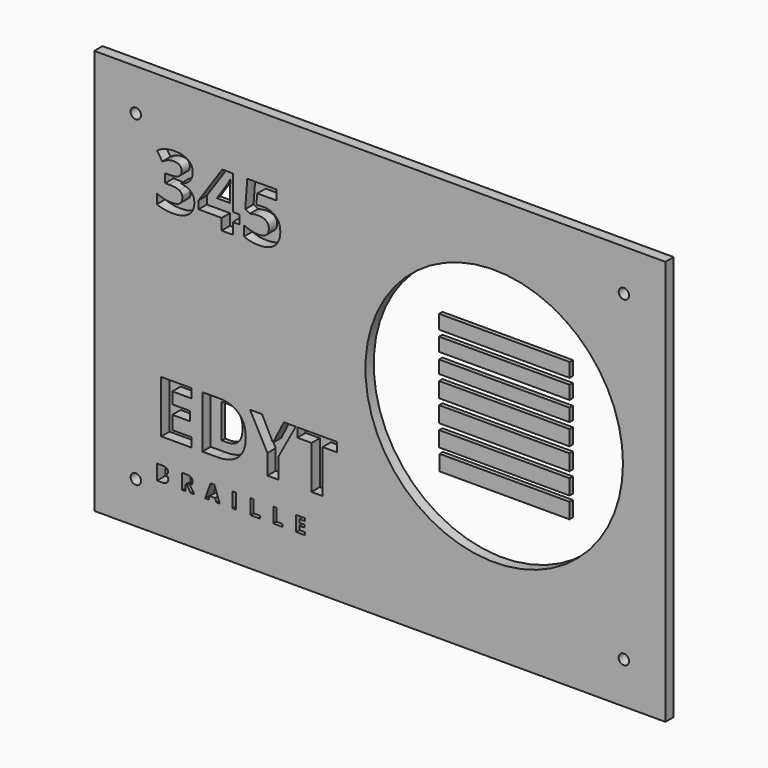
from build123d import *

# Parameters (mm, degrees)
F0_W           = 349.25
F0_H           = 247.65
F0_R           = 3.175
F0_W_2         = 1.9502034897
F0_H_2         = 9.195541532
F0_R_2         = 78.7423234547
F1_DEPTH       = 6.35
F0_W_3         = 79.7690153122
F0_H_3         = 8.5733048618
F0_H_4         = 8.2005523145
F0_H_5         = 7.8277997673
F0_H_6         = 9.3188099563
F0_H_7         = 9.6915662289
F0_H_8         = 9.3188136816
F0_W_4         = 79.3962478638
F0_H_9         = 9.4509058177
F0_TEXT_SIZE   = 44.8574507982
F0_TEXT_SIZE_2 = 46.3020833333
F2_DEPTH       = 2.54


# Not quite as in the source:
# - Text() gives the source's letters only with a copy of the font that has no kerning and outlines rounded to 1/6400 em; it was checked with that copy


with BuildPart() as f1:
    # F0 (on Front) → F1 (new body)
    with BuildSketch(Plane.XZ):
        with Locations((111.7297765017, -62.4566947639)):
            Rectangle(F0_W, F0_H)
        with Locations((-37.4952234983, -160.8816947639)):
            Circle(F0_R, mode=Mode.SUBTRACT)
        with BuildLine():
            Line((-24.4460603303, -157.455727458), (-24.4460603303, -148.260185926))
            Line((-24.4460603303, -148.260185926), (-21.5841518036, -148.260185926))
            add(Edge.make_bspline(
                [(-21.5841518036, -148.260185926), (-19.6279105322, -148.260185926), (-18.7443818098, -148.8166681395)],
                knots=[0, 0, 0, 1, 1, 1], degree=2))
            add(Edge.make_bspline(
                [(-18.7443818098, -148.8166681395), (-17.8608530874, -149.3731503531), (-17.8608530874, -150.5867444752)],
                knots=[0, 0, 0, 1, 1, 1], degree=2))
            add(Edge.make_bspline(
                [(-17.8608530874, -150.5867444752), (-17.8608530874, -151.4119079744), (-18.2472711163, -151.9402138733)],
                knots=[0, 0, 0, 1, 1, 1], degree=2))
            add(Edge.make_bspline(
                [(-18.2472711163, -151.9402138733), (-18.6336891453, -152.4685197722), (-19.2757065996, -152.575187249)],
                knots=[0, 0, 0, 1, 1, 1], degree=2))
            Line((-19.2757065996, -152.575187249), (-19.2757065996, -152.6375776599))
            add(Edge.make_bspline(
                [(-19.2757065996, -152.6375776599), (-18.4022408467, -152.8327992683), (-18.0148165208, -153.3671429489)],
                knots=[0, 0, 0, 1, 1, 1], degree=2))
            add(Edge.make_bspline(
                [(-18.0148165208, -153.3671429489), (-17.6273921949, -153.9014866295), (-17.6273921949, -154.7890405397)],
                knots=[0, 0, 0, 1, 1, 1], degree=2))
            add(Edge.make_bspline(
                [(-17.6273921949, -154.7890405397), (-17.6273921949, -156.0469117276), (-18.537084638, -156.7513195928)],
                knots=[0, 0, 0, 1, 1, 1], degree=2))
            add(Edge.make_bspline(
                [(-18.537084638, -156.7513195928), (-19.4467770811, -157.455727458), (-21.0065373541, -157.455727458)],
                knots=[0, 0, 0, 1, 1, 1], degree=2))
            Line((-21.0065373541, -157.455727458), (-24.4460603303, -157.455727458))
        make_face(mode=Mode.SUBTRACT)
        with BuildLine():
            Line((-6.1113298955, -153.9276503502), (-7.1478157544, -153.9276503502))
            Line((-7.1478157544, -153.9276503502), (-7.1478157544, -157.455727458))
            Line((-7.1478157544, -157.455727458), (-9.0980192441, -157.455727458))
            Line((-9.0980192441, -157.455727458), (-9.0980192441, -148.260185926))
            Line((-9.0980192441, -148.260185926), (-6.4192567623, -148.260185926))
            add(Edge.make_bspline(
                [(-6.4192567623, -148.260185926), (-4.543519247, -148.260185926), (-3.6448960703, -148.9424552583)],
                knots=[0, 0, 0, 1, 1, 1], degree=2))
            add(Edge.make_bspline(
                [(-3.6448960703, -148.9424552583), (-2.7462728937, -149.6247245907), (-2.7462728937, -151.015426976)],
                knots=[0, 0, 0, 1, 1, 1], degree=2))
            add(Edge.make_bspline(
                [(-2.7462728937, -151.015426976), (-2.7462728937, -151.8265023179), (-3.1920624427, -152.4584568027)],
                knots=[0, 0, 0, 1, 1, 1], degree=2))
            add(Edge.make_bspline(
                [(-3.1920624427, -152.4584568027), (-3.6378519917, -153.0904112875), (-4.4569777092, -153.4486530018)],
                knots=[0, 0, 0, 1, 1, 1], degree=2))
            add(Edge.make_bspline(
                [(-4.4569777092, -153.4486530018), (-2.3799808038, -156.5500602027), (-1.7520515068, -157.455727458)],
                knots=[0, 0, 0, 1, 1, 1], degree=2))
            Line((-1.7520515068, -157.455727458), (-3.91558995, -157.455727458))
            Line((-3.91558995, -157.455727458), (-6.1113298955, -153.9276503502))
        make_face(mode=Mode.SUBTRACT)
        Polygon((13.8294504719, -157.455727458), (11.7283024396, -157.455727458), (11.0621338585, -155.2660252941), (7.7091524201, -155.2660252941), (7.042983839, -157.455727458), (4.9418358067, -157.455727458), (8.1881497684, -148.2219466419), (10.5710609468, -148.2219466419), align=None, mode=Mode.SUBTRACT)
        with Locations((22.6556810231, -152.857956692)):
            Rectangle(F0_W_2, F0_H_2, mode=Mode.SUBTRACT)
        Polygon((38.3186930548, -157.455727458), (32.6391530672, -157.455727458), (32.6391530672, -148.260185926), (34.5893565569, -148.260185926), (34.5893565569, -155.8456523375), (38.3186930548, -155.8456523375), align=None, mode=Mode.SUBTRACT)
        Polygon((52.2901199129, -157.455727458), (46.6105799254, -157.455727458), (46.6105799254, -148.260185926), (48.5607834151, -148.260185926), (48.5607834151, -155.8456523375), (52.2901199129, -155.8456523375), align=None, mode=Mode.SUBTRACT)
        Polygon((65.8771413361, -155.8456523375), (65.8771413361, -157.455727458), (60.5820067835, -157.455727458), (60.5820067835, -148.260185926), (65.8771413361, -148.260185926), (65.8771413361, -149.8581854831), (62.5322102732, -149.8581854831), (62.5322102732, -151.8768171655), (65.6456930375, -151.8768171655), (65.6456930375, -153.4748167226), (62.5322102732, -153.4748167226), (62.5322102732, -155.8456523375), align=None, mode=Mode.SUBTRACT)
        Polygon((-3.5052732486, -127.2468779888), (-3.5052732486, -132.8540593386), (-21.9458909126, -132.8540593386), (-21.9458909126, -100.8300448547), (-3.5052732486, -100.8300448547), (-3.5052732486, -106.3951723443), (-15.1541925027, -106.3951723443), (-15.1541925027, -113.4251759616), (-4.3113055676, -113.4251759616), (-4.3113055676, -118.9903034513), (-15.1541925027, -118.9903034513), (-15.1541925027, -127.2468779888), align=None, mode=Mode.SUBTRACT)
        with BuildLine():
            add(Edge.make_bspline(
                [(25.4067555862, -104.9688455885), (29.7453121556, -109.1076463223), (29.7453121556, -116.5371616107)],
                knots=[0, 0, 0, 1, 1, 1], degree=2))
            add(Edge.make_bspline(
                [(29.7453121556, -116.5371616107), (29.7453121556, -124.4432873139), (25.242044634, -128.6486733262)],
                knots=[0, 0, 0, 1, 1, 1], degree=2))
            add(Edge.make_bspline(
                [(25.242044634, -128.6486733262), (20.7387771125, -132.8540593386), (12.2438973676, -132.8540593386)],
                knots=[0, 0, 0, 1, 1, 1], degree=2))
            Line((12.2438973676, -132.8540593386), (3.1742815344, -132.8540593386))
            Line((3.1742815344, -132.8540593386), (3.1742815344, -100.8300448547))
            Line((3.1742815344, -100.8300448547), (13.2251541038, -100.8300448547))
            add(Edge.make_bspline(
                [(13.2251541038, -100.8300448547), (21.0681990168, -100.8300448547), (25.4067555862, -104.9688455885)],
                knots=[0, 0, 0, 1, 1, 1], degree=2))
        make_face(mode=Mode.SUBTRACT)
        Polygon((39.7120770048, -100.8300448547), (46.3495779276, -114.0139300033), (53.0291327105, -100.8300448547), (60.3465043719, -100.8300448547), (49.7208957141, -120.3920987887), (49.7208957141, -132.8540593386), (42.978260141, -132.8540593386), (42.978260141, -120.609377066), (32.3526514832, -100.8300448547), align=None, mode=Mode.SUBTRACT)
        Polygon((76.7334918666, -106.4792800646), (76.7334918666, -132.8540593386), (69.9417934567, -132.8540593386), (69.9417934567, -106.4792800646), (61.2436533879, -106.4792800646), (61.2436533879, -100.8300448547), (85.4246229588, -100.8300448547), (85.4246229588, -106.4792800646), align=None, mode=Mode.SUBTRACT)
        with Locations((260.9547765017, -160.8816947639)):
            Circle(F0_R, mode=Mode.SUBTRACT)
        with BuildLine():
            add(Edge.make_bspline(
                [(-5.6503231396, 21.3764310499), (-2.6768612256, 19.2964546502), (-2.6768612256, 15.5922879835)],
                knots=[0, 0, 0, 1, 1, 1], degree=2))
            add(Edge.make_bspline(
                [(-2.6768612256, 15.5922879835), (-2.6768612256, 12.4958361606), (-4.5542660107, 10.3254260043)],
                knots=[0, 0, 0, 1, 1, 1], degree=2))
            add(Edge.make_bspline(
                [(-4.5542660107, 10.3254260043), (-6.4316707959, 8.1550158481), (-9.8247453401, 7.3374946892)],
                knots=[0, 0, 0, 1, 1, 1], degree=2))
            Line((-9.8247453401, 7.3374946892), (-9.8247453401, 7.2072700799))
            add(Edge.make_bspline(
                [(-9.8247453401, 7.2072700799), (-5.8167212516, 6.7080757439), (-3.7620663037, 4.7727933546)],
                knots=[0, 0, 0, 1, 1, 1], degree=2))
            add(Edge.make_bspline(
                [(-3.7620663037, 4.7727933546), (-1.7074113558, 2.8375109653), (-1.7074113558, -0.4398083707)],
                knots=[0, 0, 0, 1, 1, 1], degree=2))
            add(Edge.make_bspline(
                [(-1.7074113558, -0.4398083707), (-1.7074113558, -5.2074760139), (-5.1655982047, -7.8662284553)],
                knots=[0, 0, 0, 1, 1, 1], degree=2))
            add(Edge.make_bspline(
                [(-5.1655982047, -7.8662284553), (-8.6237850537, -10.5249808967), (-15.0409644157, -10.5249808967)],
                knots=[0, 0, 0, 1, 1, 1], degree=2))
            add(Edge.make_bspline(
                [(-15.0409644157, -10.5249808967), (-20.4235816032, -10.5249808967), (-24.5835344026, -8.7380098681)],
                knots=[0, 0, 0, 1, 1, 1], degree=2))
            Line((-24.5835344026, -8.7380098681), (-24.5835344026, -2.7910860399))
            add(Edge.make_bspline(
                [(-24.5835344026, -2.7910860399), (-22.6663387646, -3.7605359097), (-20.3584692985, -4.3718681037)],
                knots=[0, 0, 0, 1, 1, 1], degree=2))
            add(Edge.make_bspline(
                [(-20.3584692985, -4.3718681037), (-18.0505998323, -4.9832002978), (-15.7933732698, -4.9832002978)],
                knots=[0, 0, 0, 1, 1, 1], degree=2))
            add(Edge.make_bspline(
                [(-15.7933732698, -4.9832002978), (-12.3279517204, -4.9832002978), (-10.6784400016, -3.8075614631)],
                knots=[0, 0, 0, 1, 1, 1], degree=2))
            add(Edge.make_bspline(
                [(-10.6784400016, -3.8075614631), (-9.0289282829, -2.6319226285), (-9.0289282829, -0.027430441)],
                knots=[0, 0, 0, 1, 1, 1], degree=2))
            add(Edge.make_bspline(
                [(-9.0289282829, -0.027430441), (-9.0289282829, 2.2949084262), (-10.9280371696, 3.2679756463)],
                knots=[0, 0, 0, 1, 1, 1], degree=2))
            add(Edge.make_bspline(
                [(-10.9280371696, 3.2679756463), (-12.8271460563, 4.2410428663), (-16.9870988558, 4.2410428663)],
                knots=[0, 0, 0, 1, 1, 1], degree=2))
            Line((-16.9870988558, 4.2410428663), (-19.4975399365, 4.2410428663))
            Line((-19.4975399365, 4.2410428663), (-19.4975399365, 9.6019559522))
            Line((-19.4975399365, 9.6019559522), (-16.9436906526, 9.6019559522))
            add(Edge.make_bspline(
                [(-16.9436906526, 9.6019559522), (-13.1020646761, 9.6019559522), (-11.3259456982, 10.6075793246)],
                knots=[0, 0, 0, 1, 1, 1], degree=2))
            add(Edge.make_bspline(
                [(-11.3259456982, 10.6075793246), (-9.5498267204, 11.613202697), (-9.5498267204, 14.0512967726)],
                knots=[0, 0, 0, 1, 1, 1], degree=2))
            add(Edge.make_bspline(
                [(-9.5498267204, 14.0512967726), (-9.5498267204, 17.8061063429), (-14.2523820589, 17.8061063429)],
                knots=[0, 0, 0, 1, 1, 1], degree=2))
            add(Edge.make_bspline(
                [(-14.2523820589, 17.8061063429), (-15.8801896761, 17.8061063429), (-17.5658748974, 17.2635038038)],
                knots=[0, 0, 0, 1, 1, 1], degree=2))
            add(Edge.make_bspline(
                [(-17.5658748974, 17.2635038038), (-19.2515601188, 16.7209012647), (-21.3062150667, 15.3897163689)],
                knots=[0, 0, 0, 1, 1, 1], degree=2))
            Line((-21.3062150667, 15.3897163689), (-24.5401261995, 20.2007922153))
            add(Edge.make_bspline(
                [(-24.5401261995, 20.2007922153), (-20.018438374, 23.4564074496), (-13.753187723, 23.4564074496)],
                knots=[0, 0, 0, 1, 1, 1], degree=2))
            add(Edge.make_bspline(
                [(-13.753187723, 23.4564074496), (-8.6237850537, 23.4564074496), (-5.6503231396, 21.3764310499)],
                knots=[0, 0, 0, 1, 1, 1], degree=2))
        make_face(mode=Mode.SUBTRACT)
        Polygon((25.7844506234, 2.20809202), (25.7844506234, -3.2179333707), (21.8053653369, -3.2179333707), (21.8053653369, -10.0691947639), (14.9758080453, -10.0691947639), (14.9758080453, -3.2179333707), (0.8681420296, -3.2179333707), (0.8681420296, 1.6437853793), (15.3664818734, 22.9861519158), (21.8053653369, 22.9861519158), (21.8053653369, 2.20809202), align=None, mode=Mode.SUBTRACT)
        with Locations((-37.4952234983, 35.9683052361)):
            Circle(F0_R, mode=Mode.SUBTRACT)
        with BuildLine():
            add(Edge.make_bspline(
                [(36.9765323291, 10.7305692335), (38.3583601286, 11.0488960564), (40.391310975, 11.0488960564)],
                knots=[0, 0, 0, 1, 1, 1], degree=2))
            add(Edge.make_bspline(
                [(40.391310975, 11.0488960564), (45.1806827197, 11.0488960564), (48.0203026742, 8.3575874627)],
                knots=[0, 0, 0, 1, 1, 1], degree=2))
            add(Edge.make_bspline(
                [(48.0203026742, 8.3575874627), (50.8599226286, 5.6662788689), (50.8599226286, 0.9854276319)],
                knots=[0, 0, 0, 1, 1, 1], degree=2))
            add(Edge.make_bspline(
                [(50.8599226286, 0.9854276319), (50.8599226286, -4.5491182665), (47.4451439828, -7.5370495816)],
                knots=[0, 0, 0, 1, 1, 1], degree=2))
            add(Edge.make_bspline(
                [(47.4451439828, -7.5370495816), (44.0303653369, -10.5249808967), (37.6782982796, -10.5249808967)],
                knots=[0, 0, 0, 1, 1, 1], degree=2))
            add(Edge.make_bspline(
                [(37.6782982796, -10.5249808967), (32.1582217822, -10.5249808967), (28.7723819385, -8.7380098681)],
                knots=[0, 0, 0, 1, 1, 1], degree=2))
            Line((28.7723819385, -8.7380098681), (28.7723819385, -2.6970349332))
            add(Edge.make_bspline(
                [(28.7723819385, -2.6970349332), (30.5521182666, -3.6447807014), (32.9287173877, -4.2452608446)],
                knots=[0, 0, 0, 1, 1, 1], degree=2))
            add(Edge.make_bspline(
                [(32.9287173877, -4.2452608446), (35.3053165088, -4.8457409879), (37.4250837614, -4.8457409879)],
                knots=[0, 0, 0, 1, 1, 1], degree=2))
            add(Edge.make_bspline(
                [(37.4250837614, -4.8457409879), (43.8277937224, -4.8457409879), (43.8277937224, 0.3994168897)],
                knots=[0, 0, 0, 1, 1, 1], degree=2))
            add(Edge.make_bspline(
                [(43.8277937224, 0.3994168897), (43.8277937224, 5.3985949496), (37.2008080453, 5.3985949496)],
                knots=[0, 0, 0, 1, 1, 1], degree=2))
            add(Edge.make_bspline(
                [(37.2008080453, 5.3985949496), (36.0070824593, 5.3985949496), (34.5601423552, 5.1598498325)],
                knots=[0, 0, 0, 1, 1, 1], degree=2))
            add(Edge.make_bspline(
                [(34.5601423552, 5.1598498325), (33.113202251, 4.9211047153), (32.2088646859, 4.6461860955)],
                knots=[0, 0, 0, 1, 1, 1], degree=2))
            Line((32.2088646859, 4.6461860955), (29.4235049854, 6.1437691033))
            Line((29.4235049854, 6.1437691033), (30.667873475, 22.9861519158))
            Line((30.667873475, 22.9861519158), (48.5954613656, 22.9861519158))
            Line((48.5954613656, 22.9861519158), (48.5954613656, 17.0609321892))
            Line((48.5954613656, 17.0609321892), (36.7956648161, 17.0609321892))
            Line((36.7956648161, 17.0609321892), (36.1879499724, 10.571405822))
            Line((36.1879499724, 10.571405822), (36.9765323291, 10.7305692335))
        make_face(mode=Mode.SUBTRACT)
        with Locations((181.6470623016, -55.6943193078)):
            Circle(F0_R_2, mode=Mode.SUBTRACT)
        with Locations((260.9547765017, 35.9683052361)):
            Circle(F0_R, mode=Mode.SUBTRACT)
    extrude(amount=F1_DEPTH)


with BuildPart() as f2:
    # F0 (on Front) → F2 (new body)
    with BuildSketch(Plane.XZ):
        with Locations((182.7652901411, -20.0964603573)):
            Rectangle(F0_W_3, F0_H_3)
        with Locations((182.7652901411, -32.2109144181)):
            Rectangle(F0_W_3, F0_H_4)
        with Locations((182.7652901411, -44.3253684789)):
            Rectangle(F0_W_3, F0_H_5)
        with Locations((182.7652901411, -56.626195088)):
            Rectangle(F0_W_3, F0_H_6)
        with Locations((182.7652901411, -69.8589086533)):
            Rectangle(F0_W_3, F0_H_7)
        with Locations((182.7652901411, -83.0916166306)):
            Rectangle(F0_W_3, F0_H_8)
        with Locations((182.9516738653, -95.831241855)):
            Rectangle(F0_W_4, F0_H_9)
        with Locations((-25.9760525078, -132.8540593386)):
            Text('EDYT', F0_TEXT_SIZE, font='Open Sans', font_style=FontStyle.BOLD, text_align=(TextAlign.LEFT, TextAlign.BOTTOM))
        with Locations((-26.3488013297, -10.0691947639)):
            Text('345', F0_TEXT_SIZE_2, font='Open Sans', font_style=FontStyle.BOLD, text_align=(TextAlign.LEFT, TextAlign.BOTTOM))
    extrude(amount=-F2_DEPTH)


solid = Compound([f1.part, f2.part])
